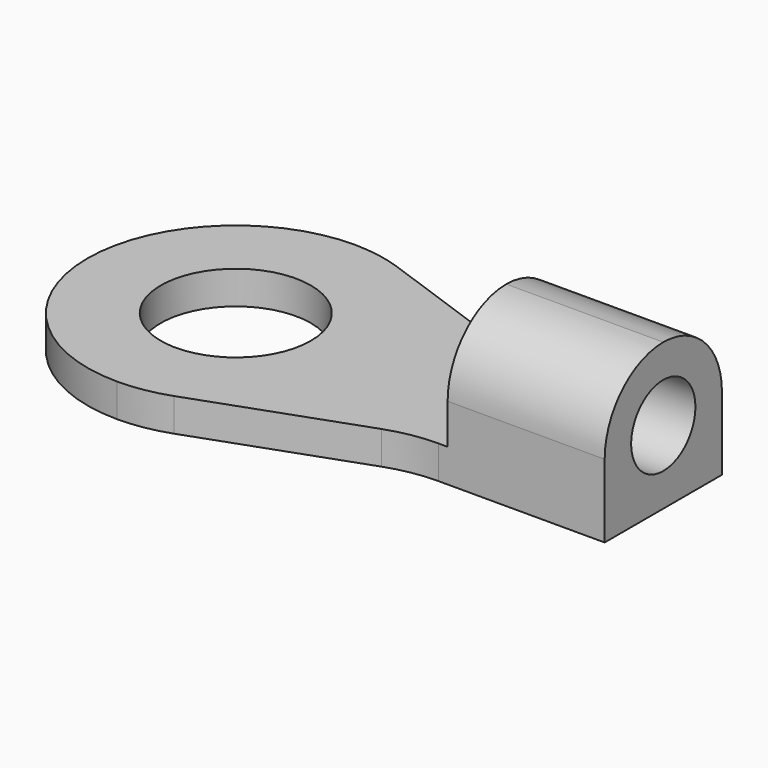
from build123d import *

# Parameters (mm, degrees)
F0_R     = 2.15
F1_DEPTH = 0.95
F2_W     = 4.5
F2_H     = 4.2
F3_DEPTH = 3.25
F4_R     = 2.09999
F5_R     = 1.15
F6_DEPTH = 25


# Not quite as in the source:
# - a fillet or chamfer is up to 0.001 mm smaller than in the source, because OpenCascade refuses the exact size


with BuildPart() as f1:
    # F0 (on Top) → F1 (new body)
    with BuildSketch(Plane.XY):
        with BuildLine():
            Line((11.7369609115, 2.15), (16.5, 2.15))
            Line((16.5, 2.15), (16.5, 6.35))
            Line((16.5, 6.35), (11.7369609115, 6.35))
            ThreePointArc((11.7369609115, 6.35), (11.0108358761, 6.4124897095), (10.306063943, 6.598121208))
            Line((10.306063943, 6.598121208), (5.6808969684, 8.251878792))
            ThreePointArc((5.6808969684, 8.251878792), (4.9761250354, 8.4375102905), (4.25, 8.5))
            ThreePointArc((4.25, 8.5), (1.24479618, 7.25520382), (0, 4.25))
            ThreePointArc((0, 4.25), (1.24479618, 1.24479618), (4.25, 0))
            ThreePointArc((4.25, 0), (4.9761250354, 0.0624897095), (5.6808969684, 0.248121208))
            Line((5.6808969684, 0.248121208), (10.306063943, 1.901878792))
            ThreePointArc((10.306063943, 1.901878792), (11.0108358761, 2.0875102905), (11.7369609115, 2.15))
        make_face()
        with Locations((4.25, 4.25)):
            Circle(F0_R, mode=Mode.SUBTRACT)
    extrude(amount=F1_DEPTH)

    # F2 (on face) → F3 (join)
    with BuildSketch(Plane.XY.offset(0.95)):
        with Locations((14.25, 4.25)):
            Rectangle(F2_W, F2_H)
    extrude(amount=F3_DEPTH)

    # F4 (radius 2.1 in the source; OpenCascade refuses exactly that, so slightly less here)
    f4_edges = [f1.edges().sort_by_distance(p)[0] for p in [
        (14.25, 6.35, 4.2),
        (14.25, 2.15, 4.2),
    ]]
    fillet(f4_edges, radius=F4_R)

    # F5 (on face) → F6 (cut)
    with BuildSketch(Plane.YZ.offset(16.5)):
        with Locations((4.25, 2.1)):
            Circle(F5_R)
    extrude(amount=-F6_DEPTH, mode=Mode.SUBTRACT)


solid = f1.part
